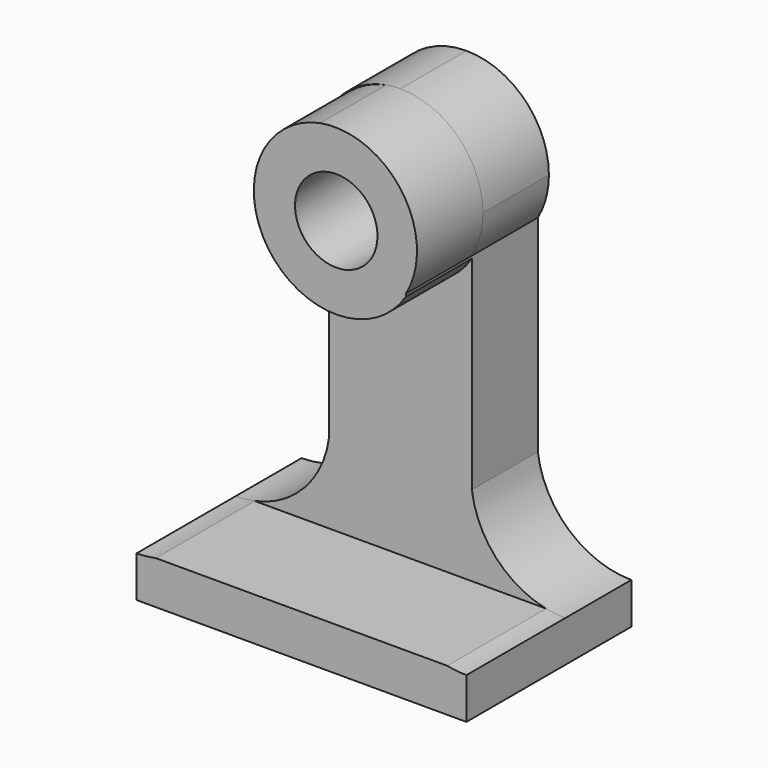
from build123d import *

# Parameters (mm, degrees)
F1_DEPTH = 12.7
F4_DEPTH = 19.05
F6_DEPTH = 12.7
F7_R     = 6.35
F8_DEPTH = 110.49


with BuildPart() as f1:
    # F0 (on Front) → F1 (new body)
    with BuildSketch(Plane.XZ):
        with BuildLine():
            ThreePointArc((27.7772603229, 13.5966521085), (24.0575164439, 22.5769082296), (15.0772603229, 26.2966521085))
            ThreePointArc((15.0772603229, 26.2966521085), (4.0787376948, 19.9466521085), (4.0787376948, 7.2466521085))
            ThreePointArc((4.0787376948, 7.2466521085), (15.0772603229, 0.8966521085), (26.0757829509, 7.2466521085))
            ThreePointArc((26.0757829509, 7.2466521085), (27.3445183167, 10.3096502357), (27.7772603229, 13.5966521085))
        make_face()
        with BuildLine():
            Line((4.0787376948, -24.5033478915), (4.0787376948, -37.2033478915))
            Line((4.0787376948, -37.2033478915), (26.0757829509, -37.2033478915))
            Line((26.0757829509, -37.2033478915), (26.0757829509, -24.5033478915))
            Line((26.0757829509, -24.5033478915), (26.0757829509, 7.2466521085))
            ThreePointArc((26.0757829509, 7.2466521085), (15.0772603229, 0.8966521085), (4.0787376948, 7.2466521085))
            Line((4.0787376948, 7.2466521085), (4.0787376948, -24.5033478915))
        make_face()
        with BuildLine():
            Line((26.0757829509, -24.5033478915), (26.0757829509, -37.2033478915))
            Line((26.0757829509, -37.2033478915), (40.4772603229, -37.2033478915))
            ThreePointArc((40.4772603229, -37.2033478915), (30.876576096, -33.5748251672), (26.0757829509, -24.5033478915))
        make_face()
        with BuildLine():
            ThreePointArc((4.0787376948, -24.5033478915), (-0.7220554503, -33.5748251672), (-10.3227396771, -37.2033478915))
            Line((-10.3227396771, -37.2033478915), (4.0787376948, -37.2033478915))
            Line((4.0787376948, -37.2033478915), (4.0787376948, -24.5033478915))
        make_face()
        Polygon((4.0787376948, -37.2033478915), (-10.3227396771, -37.2033478915), (-10.3227396771, -43.5533478915), (40.4772603229, -43.5533478915), (40.4772603229, -37.2033478915), (26.0757829509, -37.2033478915), align=None)
    extrude(amount=F1_DEPTH)

    # F3 (on face) → F4 (join)
    with BuildSketch(Plane.XZ.offset(12.7)):
        with BuildLine():
            ThreePointArc((40.4772603229, -37.2033478915), (38.989932999, -37.1269472667), (37.5182624684, -36.8985496461))
            Line((37.5182624684, -36.8985496461), (-7.3637418227, -36.8985496461))
            ThreePointArc((-7.3637418227, -36.8985496461), (-8.8354123533, -37.1269472667), (-10.3227396771, -37.2033478915))
            Line((-10.3227396771, -37.2033478915), (-10.3227396771, -43.5533478915))
            Line((-10.3227396771, -43.5533478915), (40.4772603229, -43.5533478915))
            Line((40.4772603229, -43.5533478915), (40.4772603229, -37.2033478915))
        make_face()
    extrude(amount=F4_DEPTH)

    # F5 (on face) → F6 (join)
    with BuildSketch(Plane.XZ.offset(12.7)):
        with BuildLine():
            ThreePointArc((26.0757829509, 7.2466521085), (25.482031486, 20.8788727205), (12.8772183881, 26.1046421743))
            ThreePointArc((12.8772183881, 26.1046421743), (4.8688817883, 6.4640315912), (26.0757829509, 6.8569466568))
            Line((26.0757829509, 6.8569466568), (26.0757829509, 7.2466521085))
        make_face()
    extrude(amount=F6_DEPTH)

    # F7 (on face) → F8 (cut)
    with BuildSketch(Plane.XZ.offset(25.4)):
        with Locations((15.3429014608, 13.6462952942)):
            Circle(F7_R)
    extrude(amount=-F8_DEPTH, mode=Mode.SUBTRACT)


solid = f1.part
